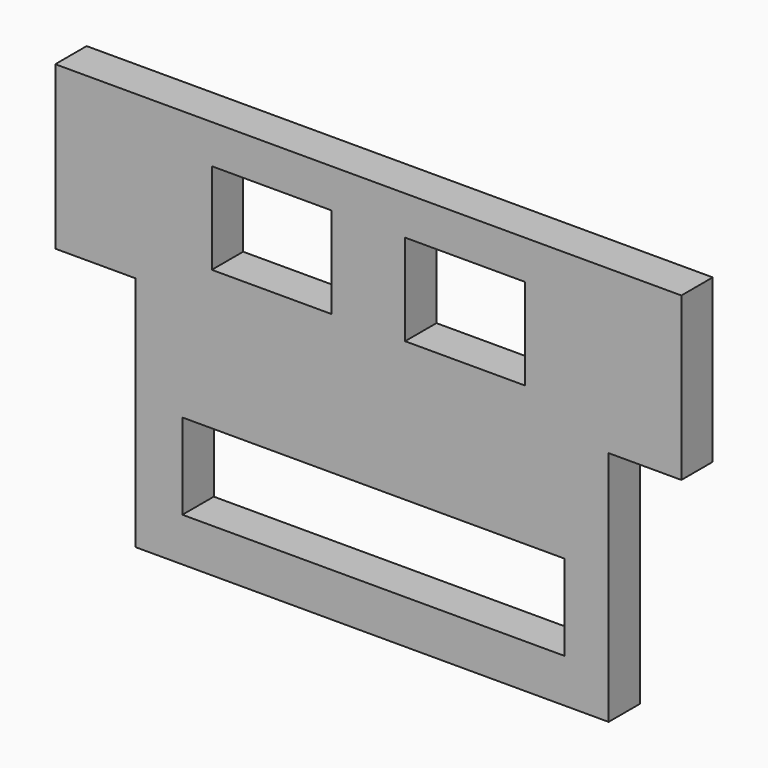
from build123d import *

# Parameters (mm, degrees)
F0_W     = 101.399846375
F0_H     = 52.6096001267
F0_W_2   = 38.787077181
F0_H_2   = 29.5493621379
F1_DEPTH = 12.7
F3_W     = 153.2556563616
F3_H     = 76.6561478376
F3_W_2   = 123.7184926867
F3_H_2   = 27.7441889048
F4_DEPTH = 12.7


# Not quite as in the source:
# - the program builds the solid bodies; features that only make, move or delete a surface that nothing else refers to are left out


with BuildPart() as f1:
    # F0 (on Front) → F1 (new body)
    with BuildSketch(Plane.XZ):
        with Locations((-50.6999231875, 26.3048000634)):
            Rectangle(F0_W, F0_H)
        with Locations((-31.306384597, 25.2366727218)):
            Rectangle(F0_W_2, F0_H_2, mode=Mode.SUBTRACT)
    extrude(amount=F1_DEPTH)

    # F2: F1 across plane


with BuildPart() as f1_1:
    add(f1.part)
    add(f1.part.mirror(Plane.YZ))

    # F3 (on Front) → F4 (join)
    with BuildSketch(Plane.XZ):
        with Locations((1.2047663331, -38.3280739188)):
            Rectangle(F3_W, F3_H)
        with Locations((1.6441084445, -48.6036911607)):
            Rectangle(F3_W_2, F3_H_2, mode=Mode.SUBTRACT)
    extrude(amount=F4_DEPTH)


solid = f1_1.part
